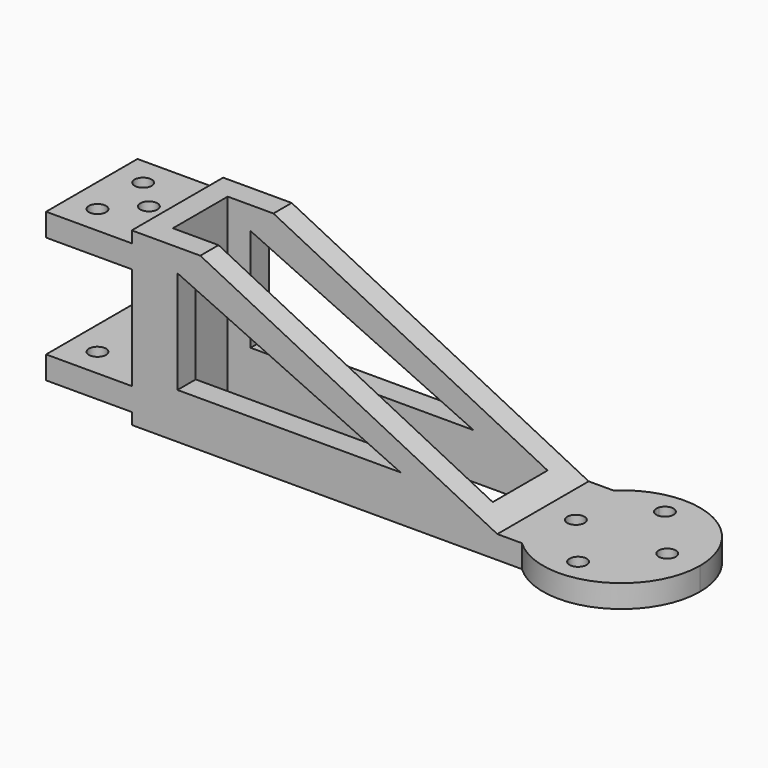
from build123d import *
from build123d import SkipClean  # not in build123d's __all__

# Parameters (mm, degrees)
F0_W        = 15
F0_H        = 4
F1_DEPTH    = 10
F2_T4_DEPTH = 20
F3_R        = 1.5
F4_DEPTH    = 4
F5_DEPTH    = 4
F7_DEPTH    = 20
F8_W        = 56
F8_H        = 12
F9_DEPTH    = 30
F10_R       = 1.5
F11_DEPTH   = 26


# Not quite as in the source:
# - a fillet or chamfer that OpenCascade refuses, or shapes differently, is made with other operations: its cross-section is extruded or revolved along the edge and cut away or added


with BuildPart() as f1:
    # F0 (on Front) → F1 (new body, symmetric)
    with BuildSketch(Plane.XZ):
        Polygon((-74.4146332145, 2), (-74.4146332145, 0), (5.5853667855, 0), (5.5853667855, 4), (-70.4146332145, 4), (-70.4146332145, 30), (-74.4146332145, 30), (-74.4146332145, 28), (-74.4146332145, 24), (-74.4146332145, 6), align=None)
        with Locations((-81.9146332145, 26)):
            Rectangle(F0_W, F0_H)
        with Locations((-81.9146332145, 4)):
            Rectangle(F0_W, F0_H)
    extrude(amount=F1_DEPTH, both=True)

    # F2: chamfer of 30 x 60 on 1 edges, made by hand


with BuildPart() as f2_tool2:
    # F2_s3 → F2_t4 (new body)
    with BuildSketch(Plane.XZ.offset(10)):
        Polygon((-70.4146332145, 34), (-10.4146332145, 4), (-70.4146332145, 4), align=None)
    extrude(amount=-F2_T4_DEPTH)

    split(bisect_by=Plane.XY.offset(30), keep=Keep.BOTTOM)


with BuildPart() as f1_1:
    add(f1.part, clean=False)

    # F2_t1: union F2_tool2
    add(f2_tool2.part)

    # F3 (on face) → F4 (join)
    with BuildSketch(Plane.XY.offset(4)):
        with BuildLine():
            ThreePointArc((-6.1019262586, -10), (8.7805353157, -12.6258718383), (17.0853667855, 0))
            ThreePointArc((17.0853667855, 0), (8.7805353157, 12.6258718383), (-6.1019262586, 10))
            Line((-6.1019262586, 10), (1.9211532232, 10))
            ThreePointArc((1.9211532232, 10), (3.3353667855, 11), (4.7495803479, 10))
            Line((4.7495803479, 10), (5.5853667855, 10))
            Line((5.5853667855, 10), (5.5853667855, -10))
            Line((5.5853667855, -10), (4.7495803479, -10))
            ThreePointArc((4.7495803479, -10), (3.3353667855, -11), (1.9211532232, -10))
            Line((1.9211532232, -10), (-6.1019262586, -10))
        make_face()
        with Locations((11.3353667855, 0)):
            Circle(F3_R, mode=Mode.SUBTRACT)
    extrude(amount=-F4_DEPTH)

    # F3 (on face) → F5 (cut)
    with BuildSketch(Plane.XY.offset(4)):
        with Locations((-4.6646332145, 0)):
            Circle(F3_R)
        with BuildLine():
            ThreePointArc((4.8353667855, -9.5), (3.0817138174, -8.0216021605), (1.9211532232, -10))
            Line((1.9211532232, -10), (4.7495803479, -10))
            ThreePointArc((4.7495803479, -10), (4.813764625, -9.7536529681), (4.8353667855, -9.5))
        make_face()
        with BuildLine():
            Line((4.7495803479, 10), (1.9211532232, 10))
            ThreePointArc((1.9211532232, 10), (3.0817138174, 8.0216021605), (4.8353667855, 9.5))
            ThreePointArc((4.8353667855, 9.5), (4.813764625, 9.7536529681), (4.7495803479, 10))
        make_face()
    with SkipClean():  # cleaning this boolean's faces spoils the solid; the shape is the same uncleaned
        extrude(amount=-F5_DEPTH, mode=Mode.SUBTRACT)

    # F6 (on face) → F7 (cut)
    with BuildSketch(Plane.XZ.offset(10)):
        Polygon((-27.3589051245, 8), (-66.4146332145, 26), (-66.4146332145, 8), align=None)
    extrude(amount=-F7_DEPTH, mode=Mode.SUBTRACT)

    # F8 (on face) → F9 (cut)
    with BuildSketch(Plane(origin=(0, 0, 0), x_dir=(1, 0, 0), z_dir=(0, 0, -1))):
        with Locations((-42.4146332145, 0)):
            Rectangle(F8_W, F8_H)
    extrude(amount=-F9_DEPTH, mode=Mode.SUBTRACT)

    # F10 (on face) → F11 (cut)
    with BuildSketch(Plane.XY.offset(28)):
        with Locations((-84.4146332145, 5)):
            Circle(F10_R)
        with Locations((-84.4146332145, -5)):
            Circle(F10_R)
        with Locations((-79.4146332145, 0)):
            Circle(F10_R)
    extrude(amount=-F11_DEPTH, mode=Mode.SUBTRACT)


solid = f1_1.part
